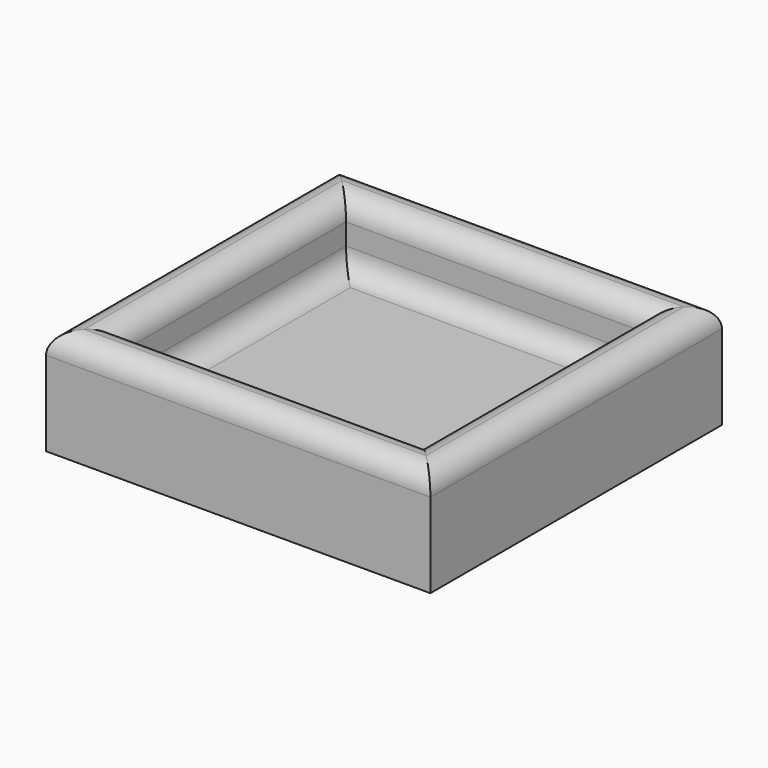
from build123d import *

# Parameters (mm, degrees)
F0_W     = 92.3412963748
F0_H     = 87.5617265701
F1_DEPTH = 25.4
F2_T     = -10.16
F3_R     = 5.07999


# Not quite as in the source:
# - a fillet or chamfer is up to 0.001 mm smaller than in the source, because OpenCascade refuses the exact size


with BuildPart() as f1:
    # F0 (on Top) → F1 (new body)
    with BuildSketch(Plane.XY):
        with Locations((-0.1911818981, -0.9559132159)):
            Rectangle(F0_W, F0_H)
    extrude(amount=F1_DEPTH)

    # F2
    f2_openings = [f1.faces().sort_by_distance(p)[0] for p in [
        (-0.191182, -0.955913, 25.4),
    ]]
    offset(amount=F2_T, openings=f2_openings)

    # F3 (radius 5.08 in the source; OpenCascade refuses exactly that, so slightly less here)
    f3_edges = [f1.edges().sort_by_distance(p)[0] for p in [
        (35.819466, -0.955913, 10.16),
        (-0.191182, 32.66495, 10.16),
        (-36.20183, -0.955913, 10.16),
        (-0.191182, -34.576777, 10.16),
        (45.979466, -0.955913, 25.4),
        (-0.191182, 42.82495, 25.4),
        (-46.36183, -0.955913, 25.4),
        (-0.191182, -44.736777, 25.4),
        (35.819466, -0.955913, 25.4),
        (-0.191182, -34.576777, 25.4),
        (-36.20183, -0.955913, 25.4),
        (-0.191182, 32.66495, 25.4),
    ]]
    fillet(f3_edges, radius=F3_R)


solid = f1.part
